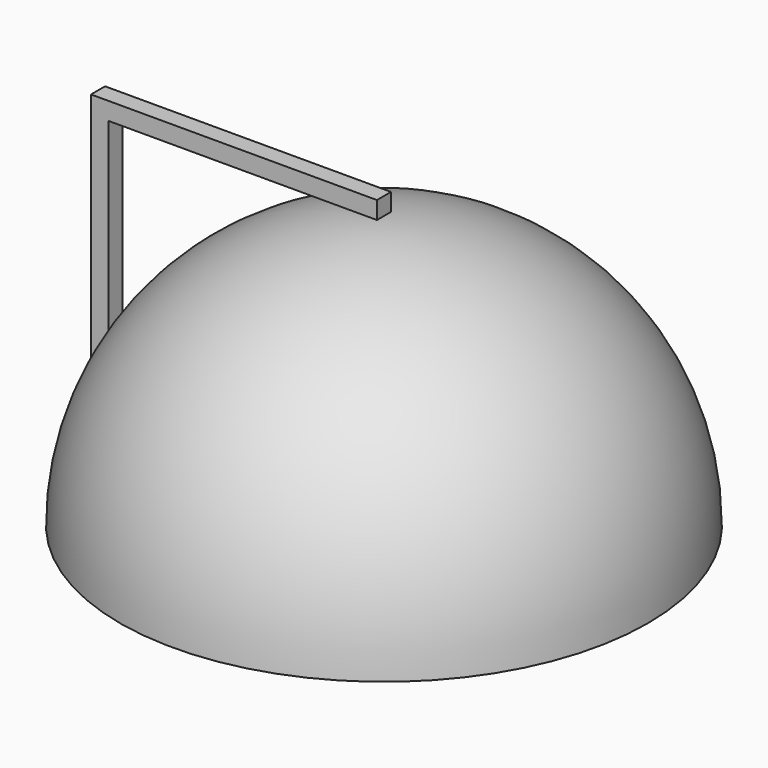
from build123d import *

# Parameters (mm, degrees)
F1_W          = 70
F1_H          = 2
F1_H_2        = 0.6
F2_W          = 4
F2_H          = 2
F2_H_2        = 58
F7_DEPTH      = 2
F7_DEPTH_BACK = 2


with BuildPart() as f3:
    # F0 (on Front) → F3 (revolve)
    with BuildSketch(Plane.XZ):
        with BuildLine():
            Line((0, 58), (0, 60))
            ThreePointArc((0, 60), (-42.4264068712, 42.4264068712), (-60, 0))
            Line((-60, 0), (-58, 0))
            ThreePointArc((-58, 0), (-41.0121933088, 41.0121933088), (0, 58))
        make_face()
    revolve(axis=Axis((0, 0, 30), (0, 0, 1)))

    # F1 (on Front) → F4 (revolve)
    with BuildSketch(Plane.XZ):
        with Locations((-35, 1)):
            Rectangle(F1_W, F1_H)
    revolve(axis=Axis((-35, 0, 0), (1, 0, 0)))

    # F1 (on Front) → F5 (revolve, cut)
    with BuildSketch(Plane.XZ):
        with Locations((-35, 2.3)):
            Rectangle(F1_W, F1_H_2)
    revolve(axis=Axis((-30, 0, 0), (-1, 0, 0)), mode=Mode.SUBTRACT)


with BuildPart() as f6:
    # F2 (on Front) → F6 (revolve)
    with BuildSketch(Plane.XZ):
        with Locations((-63, 3)):
            Rectangle(F2_W, F2_H)
    revolve(axis=Axis((-30, 0, 0), (-1, 0, 0)))

    # F2 (on Front) → F7 (join, two sides)
    with BuildSketch(Plane.XZ) as f7_sk:
        with Locations((-63, 33)):
            Rectangle(F2_W, F2_H_2)
        Polygon((-65, 62), (-61, 62), (0, 62), (0, 66), (-65, 66), align=None)
        with Locations((-63, 3)):
            Rectangle(F2_W, F2_H)
    extrude(amount=F7_DEPTH)
    extrude(f7_sk.sketch, amount=-F7_DEPTH_BACK)


solid = Compound([f3.part, f6.part])
